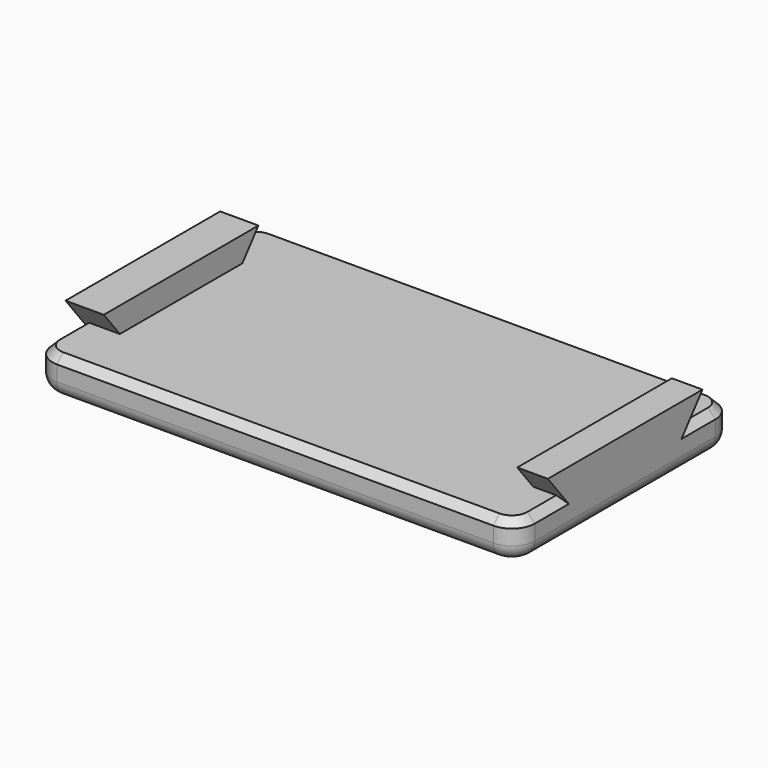
from build123d import *

# Parameters (mm, degrees)
F0_W      = 149.86
F0_H      = 80.01
F1_DEPTH  = 12.7
F0_W_2    = 160.02
F0_H_2    = 90.17
F2_DEPTH  = 12.7
F3_R      = 7.62
F4_R      = 5.08
F7_W      = 50.8
F7_H      = 6.35
F8_DEPTH  = 12.7
F9_W      = 50.8
F9_H      = 6.35
F10_DEPTH = 10.16
F11_SIZE  = 2.54


# Not quite as in the source:
# - a feature names something its author has since deleted; it is built from what else it names


with BuildPart() as f1:
    # F0 (on Top) → F1 (new body)
    with BuildSketch(Plane.XY):
        Rectangle(F0_W, F0_H)
    extrude(amount=F1_DEPTH)

    # F0 (on Top) → F2 (join)
    with BuildSketch(Plane.XY):
        Rectangle(F0_W_2, F0_H_2)
        Rectangle(F0_W, F0_H, mode=Mode.SUBTRACT)
    extrude(amount=F2_DEPTH)

    # F3
    f3_edges = [f1.edges().sort_by_distance(p)[0] for p in [
        (-80.01, 45.085, 6.35),
        (-80.01, -45.085, 6.35),
        (80.01, -45.085, 6.35),
        (80.01, 45.085, 6.35),
    ]]
    fillet(f3_edges, radius=F3_R)

    # F4
    f4_edges = [f1.edges().sort_by_distance(p)[0] for p in [
        (-80.01, 0, 0),
        (0, 45.085, 0),
        (80.01, 0, 0),
        (77.778154, 42.853154, 0),
        (77.778154, -42.853154, 0),
        (-77.778154, -42.853154, 0),
        (0, -45.085, 0),
        (-77.778154, 42.853154, 0),
    ]]
    fillet(f4_edges, radius=F4_R)

    # F7 (on face) → F8 (join)
    with BuildSketch(Plane.YZ.offset(-80.01)):
        Polygon((32.0707530211, 21.0250992866), (-32.0642467673, 21.0303084591), (-25.4, 12.7), (-25.4, 19.05), (25.4, 19.05), (25.4, 12.7), align=None)
        with Locations((0, 15.875)):
            Rectangle(F7_W, F7_H)
    extrude(amount=F8_DEPTH)

    # F9 (on face) → F10 (join)
    with BuildSketch(Plane.YZ.offset(80.01)):
        Polygon((32.0707530211, 21.0250992866), (-32.0642467673, 21.0303084591), (-25.4, 12.7), (-25.4, 19.05), (25.4, 19.05), (25.4, 12.7), align=None)
        with Locations((0, 15.875)):
            Rectangle(F9_W, F9_H)
    extrude(amount=-F10_DEPTH)

    # F11
    f11_edges = [f1.edges().sort_by_distance(p)[0] for p in [
        (0, 45.085, 12.7),
        (0, -45.085, 12.7),
        (-80.01, 31.4325, 12.7),
        (-80.01, -31.4325, 12.7),
        (-77.778154, 42.853154, 12.7),
        (-77.778154, -42.853154, 12.7),
        (77.778154, 42.853154, 12.7),
        (77.778154, -42.853154, 12.7),
        (80.01, -31.4325, 12.7),
        (80.01, 31.4325, 12.7),
    ]]
    chamfer(f11_edges, length=F11_SIZE)


solid = f1.part
